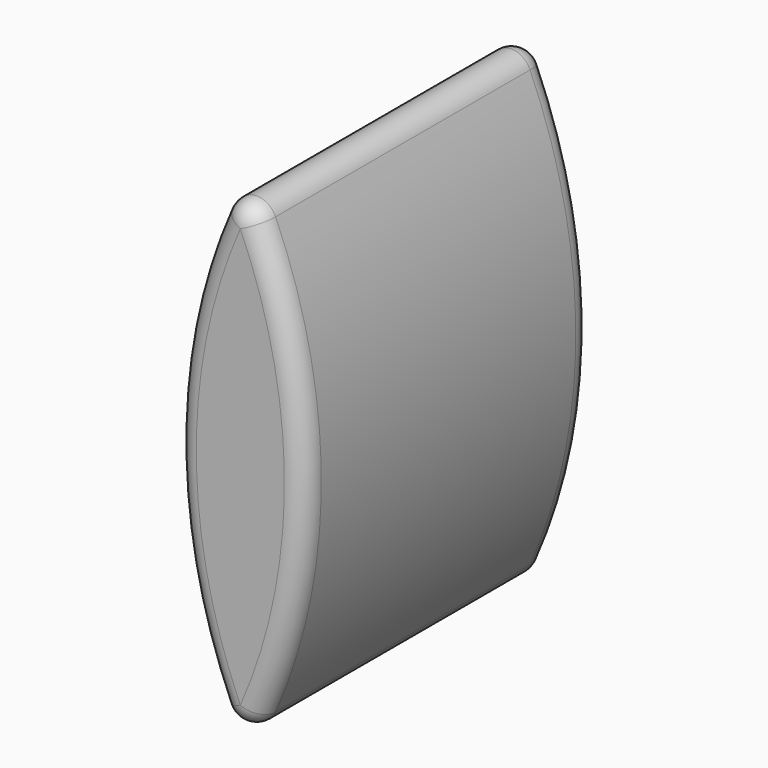
from build123d import *

# Parameters (mm, degrees)
F1_DEPTH = 88.9
F4_R     = 5.08


# Not quite as in the source:
# - a feature of the source that left no trace in its solid (it failed there, or was rolled back) is left out


with BuildPart() as f1:
    # F0 (on Front) → F1 (new body)
    with BuildSketch(Plane.XZ):
        with BuildLine():
            ThreePointArc((0, 63.2665448354), (-15.9917662052, -0.2334551646), (0, -63.7334551646))
            ThreePointArc((0, -63.7334551646), (15.9844327654, -0.2334551646), (0, 63.2665448354))
        make_face()
    extrude(amount=F1_DEPTH)

    # F4
    f4_edges = [f1.edges().sort_by_distance(p)[0] for p in [
        (0, -44.45, -63.733455),
        (0, -44.45, 63.266545),
        (15.984433, 0, -0.233455),
        (15.984433, -88.9, -0.233455),
        (-15.991766, 0, -0.233455),
        (-15.991766, -88.9, -0.233455),
    ]]
    fillet(f4_edges, radius=F4_R)


solid = f1.part
